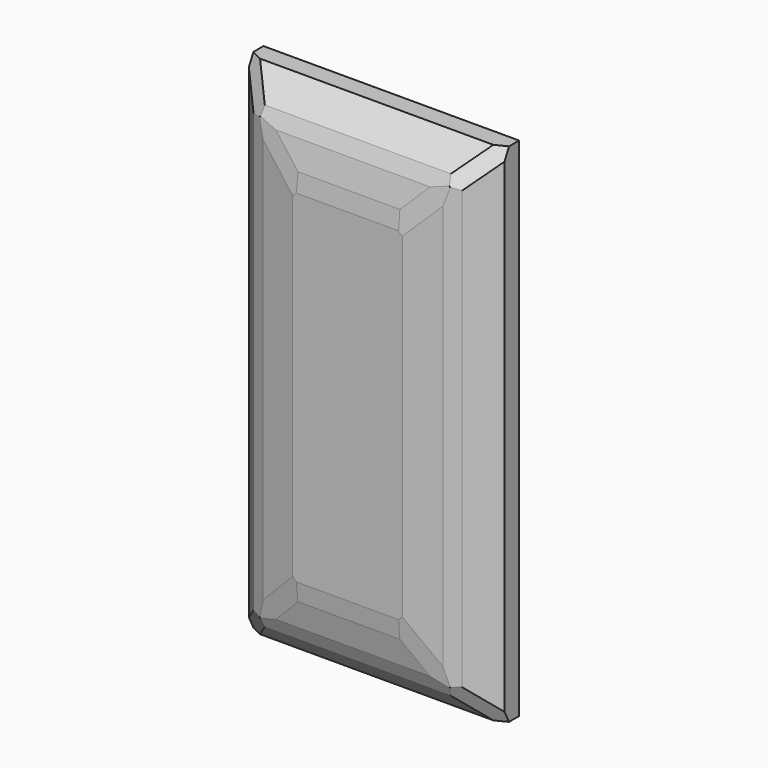
from build123d import *

# Parameters (mm, degrees)
F0_W        = 71.12
F0_H        = 140.97
F1_DEPTH    = 15.24
F2_SIZE     = 10.16
F3_SIZE     = 5.08
F4_SIZE     = 5.08
F5_SIZE     = 2.54
F6_SIZE     = 2.54
F7_T1_DEPTH = 24.5183278918
F7_T3_DEPTH = 24.5183278918
F7_T5_DEPTH = 24.5183278918
F7_T7_DEPTH = 24.5183278918


# Not quite as in the source:
# - a fillet or chamfer that OpenCascade refuses, or shapes differently, is made with other operations: its cross-section is extruded or revolved along the edge and cut away or added


with BuildPart() as f1:
    # F0 (on Front) → F1 (new body)
    with BuildSketch(Plane.XZ):
        with Locations((-1.2450981867, 23.9183327848)):
            Rectangle(F0_W, F0_H)
    extrude(amount=F1_DEPTH)

    # F2
    f2_edges = [f1.edges().sort_by_distance(p)[0] for p in [
        (-1.245098, -15.24, 94.403333),
        (34.314902, -15.24, 23.918333),
        (-36.805098, -15.24, 23.918333),
        (-1.245098, -15.24, -46.566667),
    ]]
    chamfer(f2_edges, length=F2_SIZE)

    # F3
    f3_edges = [f1.edges().sort_by_distance(p)[0] for p in [
        (-26.645098, -15.24, 23.918333),
        (-1.245098, -15.24, -36.406667),
        (24.154902, -15.24, 23.918333),
        (-1.245098, -15.24, 84.243333),
    ]]
    chamfer(f3_edges, length=F3_SIZE)

    # F4
    f4_edges = [f1.edges().sort_by_distance(p)[0] for p in [
        (-1.245098, -15.24, 79.163333),
        (-1.245098, -15.24, -31.326667),
        (-21.565098, -15.24, 23.918333),
        (19.074902, -15.24, 23.918333),
    ]]
    chamfer(f4_edges, length=F4_SIZE)

    # F5
    f5_edges = [f1.edges().sort_by_distance(p)[0] for p in [
        (18.881556, -14.267984, 78.969987),
        (-21.371752, -14.267984, 78.969987),
        (-21.371752, -14.267984, -31.133321),
        (18.881556, -14.267984, -31.133321),
    ]]
    chamfer(f5_edges, length=F5_SIZE)

    # F6
    f6_edges = [f1.edges().sort_by_distance(p)[0] for p in [
        (-1.245098, -15.24, 74.083333),
        (-1.245098, -15.24, -26.246667),
    ]]
    chamfer(f6_edges, length=F6_SIZE)

    # F7: chamfer of 2.54 on 4 edges, made by hand

    # F7_s2 → F7_t1 (cut)
    with BuildSketch(Plane(origin=(29.0610725046, 29.0610725046, -29.0610725046), x_dir=(0.7071067812, -0.7071067812, 0), z_dir=(-0.5773502692, -0.5773502692, 0.5773502692))):
        Polygon((25.6566976907, -27.3564258793), (27.8564022163, -23.5464258793), (27.8564022163, -26.0864258793), align=None)
    extrude(amount=F7_T1_DEPTH, mode=Mode.SUBTRACT)

    # F7_s4 → F7_t3 (cut)
    with BuildSketch(Plane(origin=(45.0066276944, 45.0066276944, 45.0066276944), x_dir=(0.7071067812, -0.7071067812, 0), z_dir=(-0.5773502692, -0.5773502692, -0.5773502692))):
        Polygon((27.8564022163, 62.6048997598), (25.6566976907, 66.4148997598), (27.8564022163, 65.1448997598), align=None)
    extrude(amount=F7_T3_DEPTH, mode=Mode.SUBTRACT)

    # F7_s6 → F7_t5 (cut)
    with BuildSketch(Plane(origin=(-45.8366931523, 45.8366931523, 45.8366931523), x_dir=(0.7071067812, 0.7071067812, 0), z_dir=(0.5773502692, -0.5773502692, -0.5773502692))):
        Polygon((-29.6172369585, 61.5882813474), (-27.4175324329, 65.3982813474), (-29.6172369585, 64.1282813474), align=None)
    extrude(amount=F7_T5_DEPTH, mode=Mode.SUBTRACT)

    # F7_s8 → F7_t7 (cut)
    with BuildSketch(Plane(origin=(-29.8911379624, 29.8911379624, -29.8911379624), x_dir=(0.7071067812, 0.7071067812, 0), z_dir=(0.5773502692, -0.5773502692, 0.5773502692))):
        Polygon((-27.4175324329, -26.3398074669), (-29.6172369585, -22.5298074669), (-29.6172369585, -25.0698074669), align=None)
    extrude(amount=F7_T7_DEPTH, mode=Mode.SUBTRACT)


solid = f1.part
